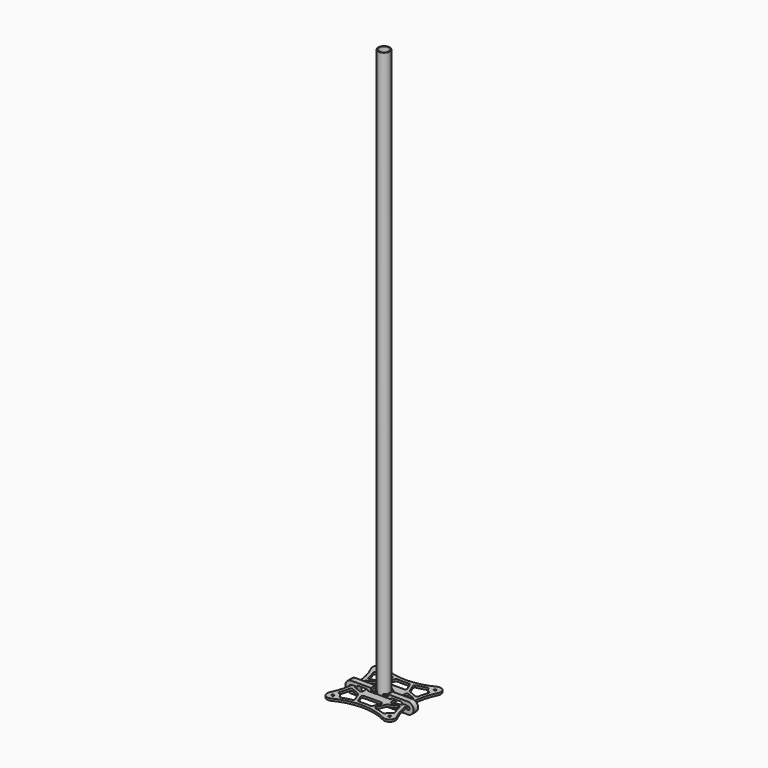
from build123d import *

# Parameters (mm, degrees)
F0_R      = 10
F0_R_2    = 9
F1_DEPTH  = 1000
F4_R      = 3.1
F4_W      = 20
F4_H      = 12
F5_DEPTH  = 10
F6_R      = 3
F7_R      = 2.1
F8_DEPTH  = 3.7
F9_R      = 3
F10_W     = 29.8
F10_H     = 10
F10_R     = 1.6
F11_DEPTH = 3.7
F13_D     = 2.5
F13_DEPTH = 8
F13_TIP   = 0.7510757738


# Not quite as in the source:
# - a feature names something its author has since deleted; it is built from what else it names


with BuildPart() as f1:
    # F0 (on Top) → F1 (new body)
    with BuildSketch(Plane.XY):
        Circle(F0_R)
        Circle(F0_R_2, mode=Mode.SUBTRACT)
    extrude(amount=F1_DEPTH)


with BuildPart() as f3:
    # F2 (on Top) → F3 (revolve)
    with BuildSketch(Plane.XY):
        Polygon((0, 4), (0, 0), (9, 0), (9, 7), (10, 7), (10, 10), (2.5, 10), (2.5, 4), align=None)
    revolve(axis=Axis((0, 2.8337724507, 0), (0, -1, 0)))


with BuildPart() as f5:
    # F4 (on Front) → F5 (new body)
    with BuildSketch(Plane.XZ):
        with BuildLine():
            Line((0, -10), (50, -10))
            ThreePointArc((50, -10), (60, 0), (50, 10))
            Line((50, 10), (15, 10))
            Line((15, 10), (15, 6.3))
            Line((15, 6.3), (5.1, 6.3))
            Line((5.1, 6.3), (5.1, -6))
            Line((5.1, -6), (0, -6))
            Line((0, -6), (-5.1, -6))
            Line((-5.1, -6), (-5.1, 6.3))
            Line((-5.1, 6.3), (-15, 6.3))
            Line((-15, 6.3), (-15, 10))
            Line((-15, 10), (-50, 10))
            ThreePointArc((-50, 10), (-60, 0), (-50, -10))
            Line((-50, -10), (0, -10))
        make_face()
        with Locations((-50, 0)):
            Circle(F4_R, mode=Mode.SUBTRACT)
        with Locations((-30, 0)):
            Rectangle(F4_W, F4_H, mode=Mode.SUBTRACT)
        with Locations((30, 0)):
            Rectangle(F4_W, F4_H, mode=Mode.SUBTRACT)
        with Locations((50, 0)):
            Circle(F4_R, mode=Mode.SUBTRACT)
    extrude(amount=F5_DEPTH)

    # F6
    f6_edges = [f5.edges().sort_by_distance(p)[0] for p in [
        (-40, -5, 6),
        (-20, -5, 6),
        (-20, -5, -6),
        (40, -5, -6),
        (-40, -5, -6),
        (20, -5, -6),
        (40, -5, 6),
        (20, -5, 6),
        (-5.1, -5, -6),
        (5.1, -5, -6),
    ]]
    fillet(f6_edges, radius=F6_R)

    # F13
    with Locations(Plane.XY.offset(6.3)):
        with Locations((-10.05, -5), (10.1, -5)):
            Hole(F13_D / 2, depth=F13_DEPTH)
            with Locations((0, 0, -(F13_DEPTH + F13_TIP / 2))):  # 118° drill point
                Cone(0, F13_D / 2, F13_TIP, mode=Mode.SUBTRACT)


with BuildPart() as f8:
    # F7 (on Top) → F8 (new body)
    with BuildSketch(Plane.XY):
        with BuildLine():
            ThreePointArc((45, 58.6602540378), (23.1227215967, 50.7014399584), (0, 48))
            ThreePointArc((0, 48), (-23.1227215967, 50.7014399584), (-45, 58.6602540378))
            ThreePointArc((-45, 58.6602540378), (-57.0710678119, 57.0710678119), (-58.6602540378, 45))
            ThreePointArc((-58.6602540378, 45), (-50.7014399584, 23.1227215967), (-48, 0))
            ThreePointArc((-48, 0), (-50.7014399584, -23.1227215967), (-58.6602540378, -45))
            ThreePointArc((-58.6602540378, -45), (-57.0710678119, -57.0710678119), (-45, -58.6602540378))
            ThreePointArc((-45, -58.6602540378), (-23.1227215967, -50.7014399584), (0, -48))
            ThreePointArc((0, -48), (23.1227215967, -50.7014399584), (45, -58.6602540378))
            ThreePointArc((45, -58.6602540378), (57.0710678119, -57.0710678119), (58.6602540378, -45))
            ThreePointArc((58.6602540378, -45), (50.7014399584, -23.1227215967), (48, 0))
            ThreePointArc((48, 0), (50.7014399584, 23.1227215967), (58.6602540378, 45))
            ThreePointArc((58.6602540378, 45), (57.0710678119, 57.0710678119), (45, 58.6602540378))
        make_face()
        with Locations((-50, -50)):
            Circle(F7_R, mode=Mode.SUBTRACT)
        with BuildLine():
            Line((-43.3898887621, -17.1342890482), (-25, -25))
            Line((-25, -25), (-17.1342890482, -43.3898887621))
            ThreePointArc((-17.1342890482, -43.3898887621), (-28.7479694312, -45.9607780251), (-40.0017489012, -49.812984053))
            ThreePointArc((-40.0017489012, -49.812984053), (-42.9289321881, -42.9289321881), (-49.812984053, -40.0017489012))
            ThreePointArc((-49.812984053, -40.0017489012), (-45.9607780251, -28.7479694312), (-43.3898887621, -17.1342890482))
        make_face(mode=Mode.SUBTRACT)
        with BuildLine():
            ThreePointArc((12, -42.679441545), (6.0096098212, -42.1699963047), (0, -42))
            ThreePointArc((0, -42), (-6.0096098212, -42.1699963047), (-12, -42.679441545))
            Line((-12, -42.679441545), (-19.5618389421, -25))
            Line((-19.5618389421, -25), (0, -25))
            Line((0, -25), (19.5618389421, -25))
            Line((19.5618389421, -25), (12, -42.679441545))
        make_face(mode=Mode.SUBTRACT)
        with Locations((50, -50)):
            Circle(F7_R, mode=Mode.SUBTRACT)
        with BuildLine():
            ThreePointArc((49.812984053, -40.0017489012), (42.9289321881, -42.9289321881), (40.0017489012, -49.812984053))
            ThreePointArc((40.0017489012, -49.812984053), (28.7479694312, -45.9607780251), (17.1342890482, -43.3898887621))
            Line((17.1342890482, -43.3898887621), (25, -25))
            Line((25, -25), (43.3898887621, -17.1342890482))
            ThreePointArc((43.3898887621, -17.1342890482), (45.9607780251, -28.7479694312), (49.812984053, -40.0017489012))
        make_face(mode=Mode.SUBTRACT)
        with BuildLine():
            ThreePointArc((-42, 0), (-42.1699963047, 6.0096098212), (-42.679441545, 12))
            Line((-42.679441545, 12), (-25, 19.5618389421))
            Line((-25, 19.5618389421), (-25, 0))
            Line((-25, 0), (-25, -19.5618389421))
            Line((-25, -19.5618389421), (-42.679441545, -12))
            ThreePointArc((-42.679441545, -12), (-42.1699963047, -6.0096098212), (-42, 0))
        make_face(mode=Mode.SUBTRACT)
        with BuildLine():
            ThreePointArc((-49.812984053, 40.0017489012), (-42.9289321881, 42.9289321881), (-40.0017489012, 49.812984053))
            ThreePointArc((-40.0017489012, 49.812984053), (-28.7479694312, 45.9607780251), (-17.1342890482, 43.3898887621))
            Line((-17.1342890482, 43.3898887621), (-25, 25))
            Line((-25, 25), (-43.3898887621, 17.1342890482))
            ThreePointArc((-43.3898887621, 17.1342890482), (-45.9607780251, 28.7479694312), (-49.812984053, 40.0017489012))
        make_face(mode=Mode.SUBTRACT)
        with Locations((-50, 50)):
            Circle(F7_R, mode=Mode.SUBTRACT)
        with BuildLine():
            Line((25, 19.5618389421), (42.679441545, 12))
            ThreePointArc((42.679441545, 12), (42.1699963047, 6.0096098212), (42, 0))
            ThreePointArc((42, 0), (42.1699963047, -6.0096098212), (42.679441545, -12))
            Line((42.679441545, -12), (25, -19.5618389421))
            Line((25, -19.5618389421), (25, 0))
            Line((25, 0), (25, 19.5618389421))
        make_face(mode=Mode.SUBTRACT)
        with BuildLine():
            ThreePointArc((-12, 42.679441545), (-6.0096098212, 42.1699963047), (0, 42))
            ThreePointArc((0, 42), (6.0096098212, 42.1699963047), (12, 42.679441545))
            Line((12, 42.679441545), (19.5618389421, 25))
            Line((19.5618389421, 25), (0, 25))
            Line((0, 25), (-19.5618389421, 25))
            Line((-19.5618389421, 25), (-12, 42.679441545))
        make_face(mode=Mode.SUBTRACT)
        with BuildLine():
            ThreePointArc((17.1342890482, 43.3898887621), (28.7479694312, 45.9607780251), (40.0017489012, 49.812984053))
            ThreePointArc((40.0017489012, 49.812984053), (42.9289321881, 42.9289321881), (49.812984053, 40.0017489012))
            ThreePointArc((49.812984053, 40.0017489012), (45.9607780251, 28.7479694312), (43.3898887621, 17.1342890482))
            Line((43.3898887621, 17.1342890482), (25, 25))
            Line((25, 25), (17.1342890482, 43.3898887621))
        make_face(mode=Mode.SUBTRACT)
        with Locations((50, 50)):
            Circle(F7_R, mode=Mode.SUBTRACT)
    extrude(amount=F8_DEPTH)

    # F9
    f9_edges = [f8.edges().sort_by_distance(p)[0] for p in [
        (-40.001749, 49.812984, 1.85),
        (-49.812984, 40.001749, 1.85),
        (-17.134289, 43.389889, 1.85),
        (-25, 25, 1.85),
        (-43.389889, 17.134289, 1.85),
        (-42.679442, -12, 1.85),
        (-49.812984, -40.001749, 1.85),
        (-40.001749, -49.812984, 1.85),
        (-42.679442, 12, 1.85),
        (-25, -25, 1.85),
        (-12, 42.679442, 1.85),
        (12, 42.679442, 1.85),
        (-25, 19.561839, 1.85),
        (19.561839, 25, 1.85),
        (43.389889, 17.134289, 1.85),
        (42.679442, -12, 1.85),
        (49.812984, -40.001749, 1.85),
        (12, -42.679442, 1.85),
        (-17.134289, -43.389889, 1.85),
        (-25, -19.561839, 1.85),
        (40.001749, -49.812984, 1.85),
        (42.679442, 12, 1.85),
        (19.561839, -25, 1.85),
        (43.389889, -17.134289, 1.85),
        (49.812984, 40.001749, 1.85),
        (40.001749, 49.812984, 1.85),
        (25, 19.561839, 1.85),
        (17.134289, 43.389889, 1.85),
        (-19.561839, -25, 1.85),
        (25, -25, 1.85),
        (-12, -42.679442, 1.85),
        (17.134289, -43.389889, 1.85),
        (25, 25, 1.85),
        (-19.561839, 25, 1.85),
        (25, -19.561839, 1.85),
        (-43.389889, -17.134289, 1.85),
    ]]
    fillet(f9_edges, radius=F9_R)


with BuildPart() as f11:
    # F10 (on Top) → F11 (new body)
    with BuildSketch(Plane.XY):
        Rectangle(F10_W, F10_H)
        with Locations((-10, 0)):
            Circle(F10_R, mode=Mode.SUBTRACT)
        with Locations((10, 0)):
            Circle(F10_R, mode=Mode.SUBTRACT)
    extrude(amount=F11_DEPTH)


solid = Compound([f1.part, f3.part, f5.part, f8.part, f11.part])
